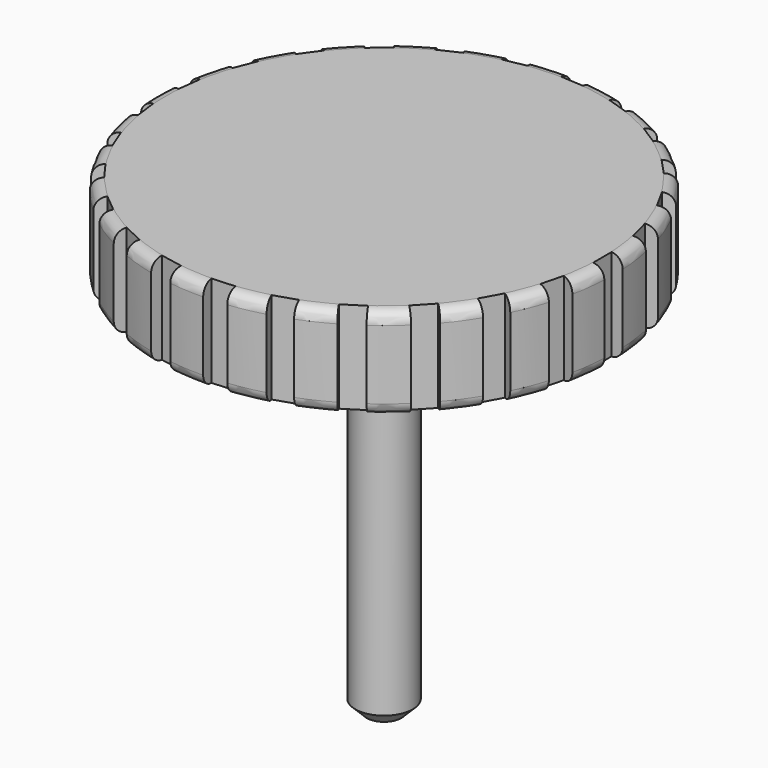
from build123d import *

# Parameters (mm, degrees)
F0_R            = 200
F1_DEPTH        = 80
F2_R            = 10
F5_W            = 20
F5_H            = 20
F6_DEPTH        = 80
F6_COPIES_COUNT = 25


# Not quite as in the source:
# - a pattern or mirror of a feature is missing from the dataset's text; its kind, count and spacing are read off the source's solid


with BuildPart() as f1:
    # F0 (on Top) → F1 (new body)
    with BuildSketch(Plane.XY):
        Circle(F0_R)
    extrude(amount=F1_DEPTH)

    # F2
    f2_edges = [f1.edges().sort_by_distance(p)[0] for p in [
        (-200, 0, 80),
        (-200, 0, 0),
    ]]
    fillet(f2_edges, radius=F2_R)

    # F3 (on Right) → F4 (revolve)
    with BuildSketch(Plane.YZ):
        Polygon((0, -330), (0, 0), (-25, 0), (-25, -320), (-15, -330), align=None)
    revolve(axis=Axis((0, 0, -165), (0, 0, -1)))

    # F5 (on face) → F6 (cut, through all)
    with BuildSketch(Plane.XY.offset(80)):
        with Locations((200, 0)):
            Rectangle(F5_W, F5_H)
    f6 = extrude(amount=-F6_DEPTH, mode=Mode.SUBTRACT)

    # F6_copies: F6 ×25 about axis
    f6_copies_axis = Axis((0, 0, 0), (0, 0, 1))
    for i in range(1, F6_COPIES_COUNT):
        add(f6.rotate(f6_copies_axis, i * 360 / F6_COPIES_COUNT), mode=Mode.SUBTRACT)


solid = f1.part
